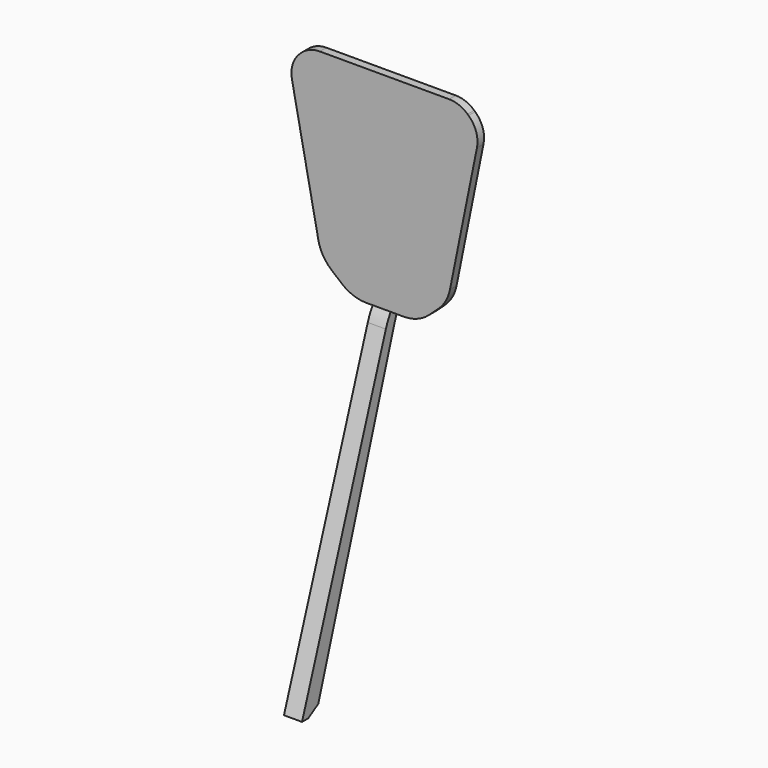
from build123d import *

# Parameters (mm, degrees)
F1_DEPTH     = 3.556
F2_R         = 12.7
F5_R         = 13.0437301263
F6_DEPTH     = 3.81
F7_R         = 12.7
F8_R         = 17.78
F10_DEPTH    = 8.382
F11_T1_DEPTH = 46.8316092758
F12_T1_DEPTH = 33.4229165443


# Not quite as in the source:
# - a fillet or chamfer that OpenCascade refuses, or shapes differently, is made with other operations: its cross-section is extruded or revolved along the edge and cut away or added
# - two fillets or chamfers of one size are made in one step


with BuildPart() as f1:
    # F0 (on Front) → F1 (new body)
    with BuildSketch(Plane.XZ):
        Polygon((-47.1675397517, 46.3941131987), (-32.3176106954, -28.3448967427), (26.3168609286, -28.3448967427), (41.4012483693, 46.3471460432), (32.0179715002, 54.9054236268), (-37.7416395402, 54.9054236268), align=None)
    extrude(amount=F1_DEPTH)

    # F2
    f2_edges = [f1.edges().sort_by_distance(p)[0] for p in [
        (-47.16754, -1.778, 46.394113),
        (41.401248, -1.778, 46.347146),
        (32.017972, -1.778, 54.905424),
        (-37.74164, -1.778, 54.905424),
    ]]
    fillet(f2_edges, radius=F2_R)

    # F5
    f5_edges = [f1.edges().sort_by_distance(p)[0] for p in [
        (26.316861, -1.778, -28.344897),
    ]]
    fillet(f5_edges, radius=F5_R)

    # F0 (on Front) → F6 (join)
    with BuildSketch(Plane.XZ):
        Polygon((26.3168609286, -28.3448967427), (-32.3176106954, -28.3448967427), (-17.7800003439, -40.6717509031), (12.8904990852, -40.6717509031), align=None)
        Polygon((-47.1675397517, 46.3941131987), (-32.3176106954, -28.3448967427), (26.3168609286, -28.3448967427), (41.4012483693, 46.3471460432), (32.0179715002, 54.9054236268), (-37.7416395402, 54.9054236268), align=None)
    extrude(amount=F6_DEPTH)

    # F7
    f7_edges = [f1.edges().sort_by_distance(p)[0] for p in [
        (32.017972, -1.905, 54.905424),
        (41.401248, -1.905, 46.347146),
        (-37.74164, -1.905, 54.905424),
        (-47.16754, -1.905, 46.394113),
    ]]
    fillet(f7_edges, radius=F7_R)

    # F8
    f8_edges = [f1.edges().sort_by_distance(p)[0] for p in [
        (-17.78, -1.905, -40.671751),
        (12.890499, -1.905, -40.671751),
        (26.316861, -1.905, -28.344897),
        (-32.317611, -1.905, -28.344897),
    ]]
    fillet(f8_edges, radius=F8_R)

    # F9 (on Right) → F10 (join)
    with BuildSketch(Plane.YZ):
        Polygon((-55.1818351742, -187.108784914), (-51.6164600849, -187.108784914), (-45.784432441, -183.5964620113), (2.1481101867, -34.6464961767), (-4.9838987179, -41.8398082256), align=None)
    extrude(amount=-F10_DEPTH)

    # F11: fillet of radius 9.6308354503 on 1 edges, made by hand

    # F11_s2 → F11_t1 (cut)
    with BuildSketch(Plane.YZ.offset(-27.6068046379)):
        with BuildLine():
            ThreePointArc((0, -36.813070433), (0.2476438249, -39.4040498919), (-0.2075604578, -41.9667225361))
            Line((-0.2075604578, -41.9667225361), (2.1481101867, -34.6464961767))
            Line((2.1481101867, -34.6464961767), (0, -36.813070433))
        make_face()
    extrude(amount=F11_T1_DEPTH, mode=Mode.SUBTRACT)

    # F12: fillet of radius 29.6825671573 on 1 edges, made by hand

    # F12_s2 → F12_t1 (cut)
    with BuildSketch(Plane.YZ.offset(-20.9024582721)):
        with BuildLine():
            ThreePointArc((-3.81, -40.6558192676), (-5.3785338271, -43.5368424871), (-6.6195826892, -46.5733521413))
            Line((-6.6195826892, -46.5733521413), (-4.9838987179, -41.8398082256))
            Line((-4.9838987179, -41.8398082256), (-3.81, -40.6558192676))
        make_face()
    extrude(amount=F12_T1_DEPTH, mode=Mode.SUBTRACT)


solid = f1.part
